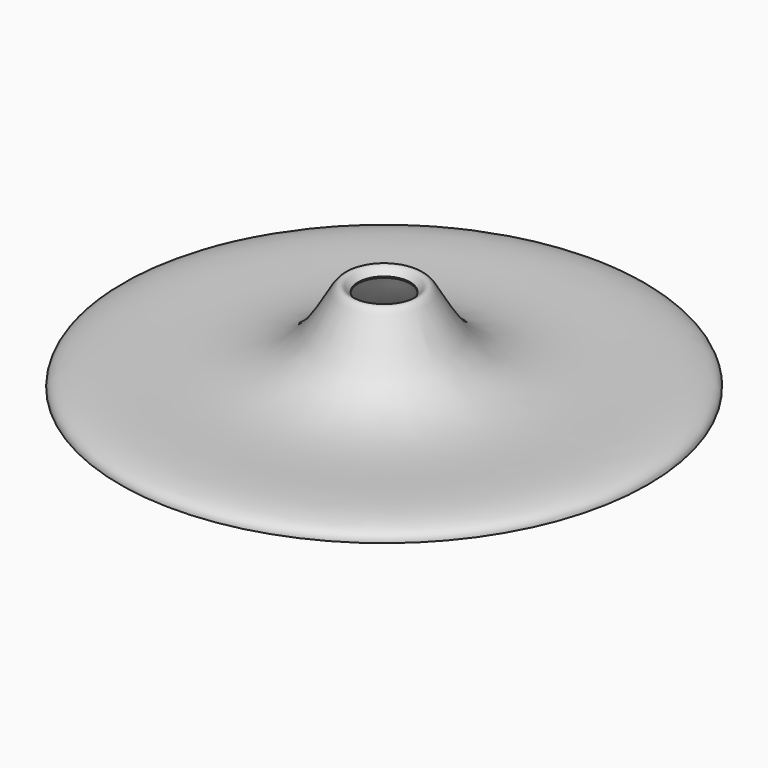
from build123d import *


with BuildPart() as f1:
    # F0 (on Front) → F1 (revolve)
    with BuildSketch(Plane.XZ):
        with BuildLine():
            add(Edge.make_bspline(
                [(15.875, 50.8254), (18.1560927399, 53.7616752819), (24.9410186921, 60.3699666141), (42.2657536287, 2.5475173788), (123.2774600612, 11.029006723), (160.1835082148, 7.373502965), (160.02, 0)],
                knots=[0, 0, 0, 0, 0.1136652529, 0.3858360884, 0.7628041128, 1, 1, 1, 1], degree=3))
            Line((15.875, 50.8254), (15.875, 50.038))
            add(Edge.make_bspline(
                [(159.22625, 0), (158.333502125, 6.6747925157), (124.0284115088, 10.3250130142), (41.9569981259, 0.5607518275), (24.4868557715, 59.3193318652), (18.6306821606, 53.4884775444), (15.875, 50.038)],
                knots=[0, 0, 0, 0, 0.2338271909, 0.6109430364, 0.8858869277, 1, 1, 1, 1], degree=3))
            Line((159.22625, 0), (160.02, 0))
        make_face()
    revolve(axis=Axis((0, 0, 25.019), (0, 0, 1)))


solid = f1.part
